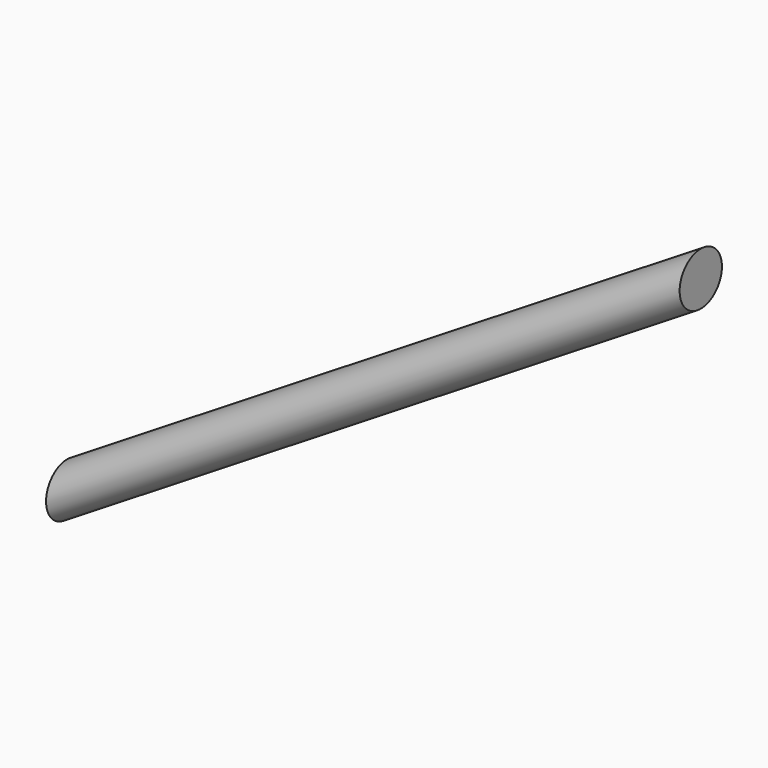
from build123d import *

# Parameters (mm, degrees)
F0_R = 10


# Not quite as in the source:
# - the program builds the solid bodies; features that only make, move or delete a surface that nothing else refers to are left out


with BuildPart() as f2:
    # F2: sweep along a path in F1
    with BuildLine(Plane.XZ) as f2_path:
        Line((0, 41.6222922504), (-239.7326529026, -106.4522638917))
    # F0 (on Right) → F2 (sweep)
    with BuildSketch(Plane.YZ):
        with Locations((0, 41.5177041402)):
            Circle(F0_R)
    sweep(path=f2_path.line)


solid = f2.part
